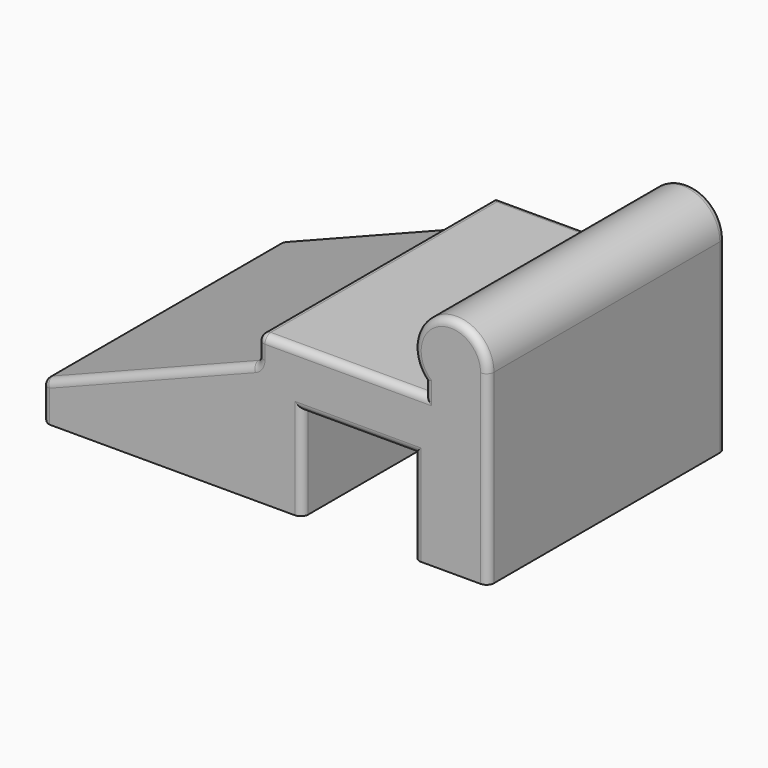
from build123d import *

# Parameters (mm, degrees)
F1_DEPTH = 80
F2_W     = 30
F2_H     = 25
F3_DEPTH = 80.001
F4_R     = 2


# Not quite as in the source:
# - a feature names something its author has since deleted; it is built from what else it names


with BuildPart() as f1:
    # F0 (on Front) → F1 (new body)
    with BuildSketch(Plane.XZ):
        with BuildLine():
            Line((112.9777067155, -18.5589175671), (112.9777067155, 31.4410824329))
            ThreePointArc((112.9777067155, 31.4410824329), (99.260783713, 40.7246422778), (95.7408100367, 24.5398270065))
            Line((95.7408100367, 24.5398270065), (95.7408100367, 21.3474755859))
            Line((95.7408100367, 21.3474755859), (50.9332562928, 21.3474755859))
            Line((50.9332562928, 21.3474755859), (50.9332562928, 14.1588503625))
            Line((50.9332562928, 14.1588503625), (-7.0222932845, -8.5589175671))
            Line((-7.0222932845, -8.5589175671), (-7.0222932845, -18.5589175671))
            Line((-7.0222932845, -18.5589175671), (112.9777067155, -18.5589175671))
        make_face()
    extrude(amount=F1_DEPTH)

    # F2 (on face) → F3 (cut, through all)
    with BuildSketch(Plane.XZ.offset(80)):
        with Locations((77.9777067155, -6.0589175671)):
            Rectangle(F2_W, F2_H)
    extrude(amount=-F3_DEPTH, mode=Mode.SUBTRACT)

    # F4
    f4_edges = [f1.edges().sort_by_distance(p)[0] for p in [
        (73.337033, -80, 21.347476),
        (95.74081, -80, 22.943651),
        (99.260784, -80, 40.724642),
        (92.977707, -80, -6.058918),
        (77.977707, -80, 6.441082),
        (62.977707, -80, -6.058918),
        (50.933256, -80, 17.753163),
        (50.933256, -40, 21.347476),
        (73.337033, 0, 21.347476),
        (-7.022293, 0, -13.558918),
        (62.977707, 0, -6.058918),
        (77.977707, 0, 6.441082),
        (92.977707, 0, -6.058918),
        (95.74081, 0, 22.943651),
        (99.260784, 0, 40.724642),
        (-7.022293, -80, -13.558918),
        (-7.022293, -40, -8.558918),
        (-7.022293, -40, -18.558918),
        (50.933256, -40, 14.15885),
        (21.955482, -80, 2.799966),
        (112.977707, 0, 6.441082),
        (112.977707, -80, 6.441082),
    ]]
    fillet(f4_edges, radius=F4_R)


solid = f1.part
